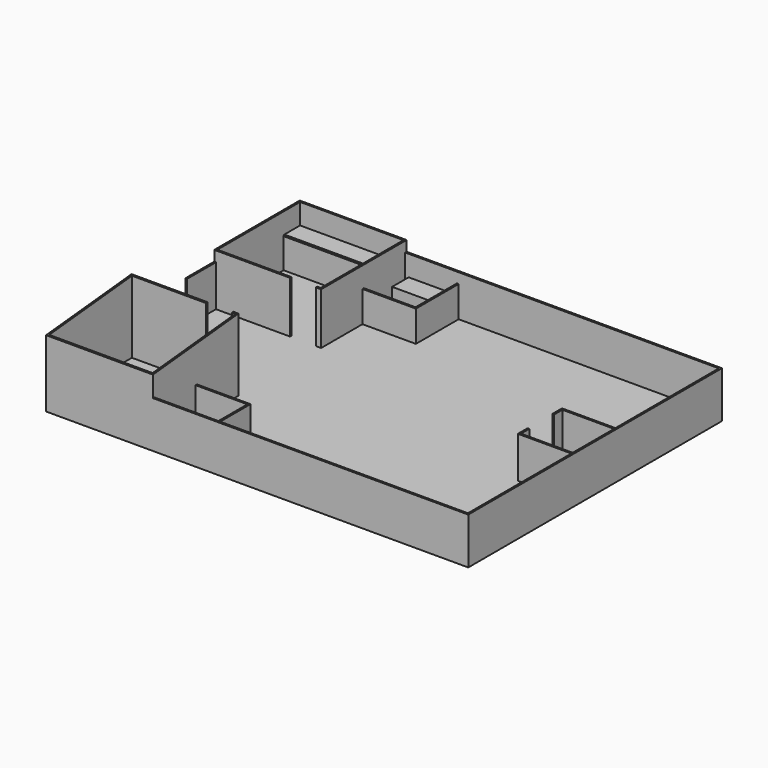
from build123d import *

# Parameters (mm, degrees)
F0_W         = 103.7166666667
F0_H         = 77.8933333333
F1_DEPTH     = 1.27
F2_W         = 102.87
F2_H         = 0.4233333333
F2_W_2       = 0.4233333333
F3_DEPTH     = 10.16
F4_W         = 25.4
F4_H         = 25.4
F5_DEPTH     = 2.54
F6_W         = 25.4
F6_H         = 5.08
F7_DEPTH     = 7.62
F8_SIZE      = 0.254
F10_DEPTH    = 17.78
F12_DEPTH    = 7.62
F14_DEPTH    = 10.16
F15_T1_DEPTH = 162.7058608064
F16_W        = 11.0460426462
F16_H        = 7.62
F16_W_2      = 6.35
F16_H_2      = 7.8945169225
F16_H_3      = 7.643327117
F17_DEPTH    = 25.4
F19_DEPTH    = 7.62
F18_R        = 0.635
F20_ANGLE    = 90
F21_W        = 8.89
F21_H        = 5.08
F22_DEPTH    = 5.08
F23_DEPTH    = 2.54


# Not quite as in the source:
# - a fillet or chamfer that OpenCascade refuses, or shapes differently, is made with other operations: its cross-section is extruded or revolved along the edge and cut away or added


with BuildPart() as f1:
    # F0 (on Top) → F1 (new body)
    with BuildSketch(Plane.XY):
        Rectangle(F0_W, F0_H)
    extrude(amount=F1_DEPTH)

    # F2 (on face) → F3 (join)
    with BuildSketch(Plane.XY.offset(1.27)):
        Polygon((-25.6116666667, 38.5233333333), (-26.035, 38.5233333333), (-26.035, 13.1233333333), (-51.435, 13.1233333333), (-51.435, 12.7), (-25.6116666667, 12.7), align=None)
        Polygon((-51.435, 13.1233333333), (-51.435, 38.5233333333), (-26.035, 38.5233333333), (-25.6116666667, 38.5233333333), (38.6280342937, 38.5233333333), (51.435, 38.5233333333), (51.8583333333, 38.5233333333), (51.8583333333, 38.9466666667), (-51.8583333333, 38.9466666667), (-51.8583333333, -38.5233333333), (-51.435, -38.5233333333), (-51.435, -30.5099412799), (-51.435, 12.7), align=None)
        Polygon((51.8583333333, 38.5233333333), (51.435, 38.5233333333), (51.435, -38.5233333333), (51.435, -38.9466666667), (51.8583333333, -38.9466666667), align=None)
        with Locations((0, -38.735)):
            Rectangle(F2_W, F2_H)
        with Locations((-51.6466666667, -38.735)):
            Rectangle(F2_W_2, F2_H)
    extrude(amount=F3_DEPTH)

    # F4 (on face) → F5 (join)
    with BuildSketch(Plane.XY.offset(11.43)):
        Polygon((-25.6116666667, 12.7), (-25.6116666667, 38.5233333333), (-25.6116666667, 38.9466666667), (-51.8583333333, 38.9466666667), (-51.8583333333, 12.7), (-51.435, 12.7), align=None)
        with Locations((-38.735, 25.8233333333)):
            Rectangle(F4_W, F4_H, mode=Mode.SUBTRACT)
    extrude(amount=F5_DEPTH)

    # F6 (on face) → F7 (join)
    with BuildSketch(Plane.XY.offset(1.27)):
        with Locations((-38.735, 35.9833333333)):
            Rectangle(F6_W, F6_H)
    extrude(amount=F7_DEPTH)

    # F8
    f8_edges = [f1.edges().sort_by_distance(p)[0] for p in [
        (-38.735, 33.443333, 8.89),
    ]]
    chamfer(f8_edges, length=F8_SIZE)

    # F9 (on face) → F10 (join)
    with BuildSketch(Plane.XY.offset(1.27)):
        Polygon((-26.035, -13.1233333333), (-26.035, -38.5233333333), (-25.6116666667, -38.5233333333), (-25.6116666667, -12.7), (-51.435, -12.7), (-51.435, -13.1233333333), align=None)
    extrude(amount=F10_DEPTH)

    # F11 (on face) → F12 (join)
    with BuildSketch(Plane.XY.offset(11.43)):
        Polygon((-25.6116666667, -38.9466666667), (-25.6116666667, -38.5233333333), (-26.035, -38.5233333333), (-51.435, -38.5233333333), (-51.435, -13.1233333333), (-51.435, -12.7), (-51.8583333333, -12.7), (-51.8583333333, -38.9466666667), align=None)
    extrude(amount=F12_DEPTH)

    # F13 (on face) → F14 (join)
    with BuildSketch(Plane.XY.offset(1.27)):
        Polygon((51.435, -6.7733333333), (51.435, -6.35), (38.735, -6.35), (38.735, -3.81), (38.3116666667, -3.81), (38.3116666667, -6.7733333333), align=None)
        Polygon((38.735, 6.35), (51.435, 6.35), (51.435, 6.7733333333), (38.3116666667, 6.7733333333), (38.3116666667, 3.81), (38.735, 3.81), align=None)
    extrude(amount=F14_DEPTH)

    # F15: chamfer of 2.54 x 26.2466666667 on 1 edges, made by hand

    # F15_s2 → F15_t1 (cut)
    with BuildSketch(Plane.YZ.offset(-120.0879304032)):
        Polygon((-12.7, 19.05), (-38.9466666667, 16.51), (-38.9466666667, 19.05), align=None)
    extrude(amount=F15_T1_DEPTH, mode=Mode.SUBTRACT)

    # F16 (on face) → F17 (cut)
    with BuildSketch(Plane.XY.offset(1.27)):
        with Locations((-51.2559060007, 0)):
            Rectangle(F16_W, F16_H)
        with Locations((-30.0566666667, 11.1596328206)):
            Rectangle(F16_W_2, F16_H_2)
        with Locations((-30.0566666667, -12.5059764832)):
            Rectangle(F16_W_2, F16_H_3)
    extrude(amount=F17_DEPTH, mode=Mode.SUBTRACT)

    # F18 (on face) → F19 (join)
    with BuildSketch(Plane.XY.offset(1.27)):
        Polygon((-12.4883333333, 38.5233333333), (-12.9116666667, 38.5233333333), (-12.9116666667, 25.8233333333), (-25.6116666667, 25.8233333333), (-25.6116666667, 25.4), (-12.4883333333, 25.4), align=None)
        Polygon((-12.9116666667, -38.5233333333), (-12.4883333333, -38.5233333333), (-12.4883333333, -25.4), (-25.6116666667, -25.4), (-25.6116666667, -25.8233333333), (-12.9116666667, -25.8233333333), align=None)
    extrude(amount=F19_DEPTH)

    # F18 (on face) → F20 (revolve)
    with BuildSketch(Plane.XY.offset(1.27)):
        with Locations((-14.3933333333, 37.0416666667)):
            Circle(F18_R)
        with Locations((-14.3933333333, -37.0416666667)):
            Circle(F18_R)
    revolve(axis=Axis((-15.4516666667, 37.5929450293, 1.27), (0, -1, 0)), revolution_arc=F20_ANGLE)

    # F21 (on face) → F22 (join)
    with BuildSketch(Plane.XY.offset(1.27)):
        with Locations((-20.32, 35.9833333333)):
            Rectangle(F21_W, F21_H)
        with Locations((-20.32, -35.9833333333)):
            Rectangle(F21_W, F21_H)
    extrude(amount=F22_DEPTH)

    # F23 (add): faces of the model
    f23_faces = [f1.faces().sort_by_distance(p)[0] for p in [
        (-15.4516666667, 37.0416666667, 2.3283333333),
        (-15.4516666667, -37.0416666667, 2.3283333333),
    ]]
    extrude(f23_faces, amount=F23_DEPTH)


solid = f1.part
